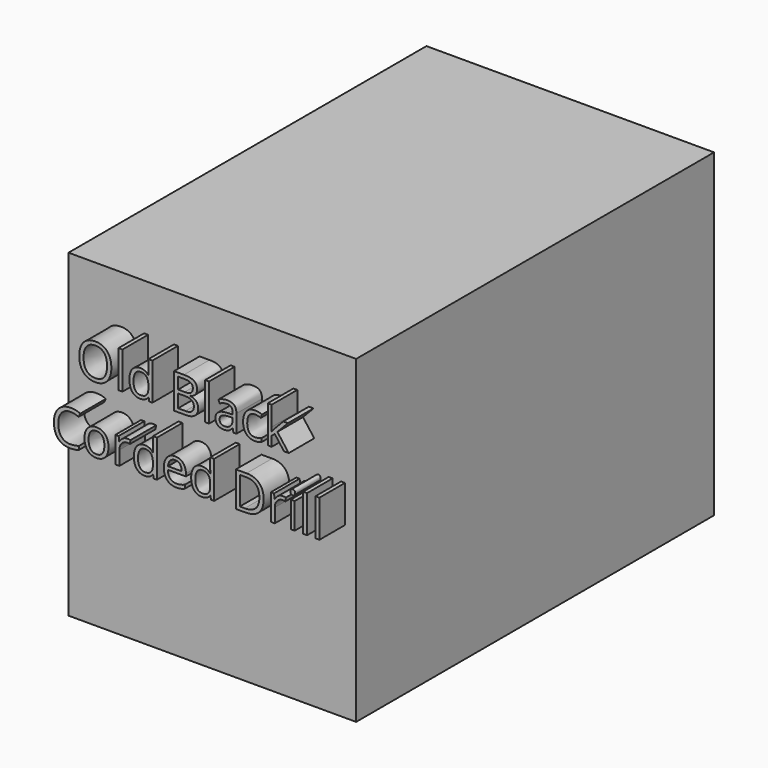
from build123d import *

# Parameters (mm, degrees)
F0_W         = 228.6
F0_H         = 254
F1_DEPTH     = 355.6
F2_TEXT_SIZE = 38.7960467206
F3_DEPTH     = 25.4


# Not quite as in the source:
# - Text() gives the source's letters only with a copy of the font that has no kerning and outlines rounded to 1/6400 em; it was checked with that copy


with BuildPart() as f1:
    # F0 (on Front) → F1 (new body)
    with BuildSketch(Plane.XZ):
        Rectangle(F0_W, F0_H)
    extrude(amount=F1_DEPTH)

    # F2 (on face) → F3 (join)
    with BuildSketch(Plane.XZ.offset(355.6)):
        with Locations((-87.7881794699, 60.6224535664)):
            Text('Old Black', F2_TEXT_SIZE, font='Open Sans', text_align=(TextAlign.LEFT, TextAlign.BOTTOM))
        with Locations((-107.95, 7.8598300264)):
            Text('Corded Drill', F2_TEXT_SIZE, font='Open Sans', text_align=(TextAlign.LEFT, TextAlign.BOTTOM))
    extrude(amount=F3_DEPTH)


solid = f1.part
